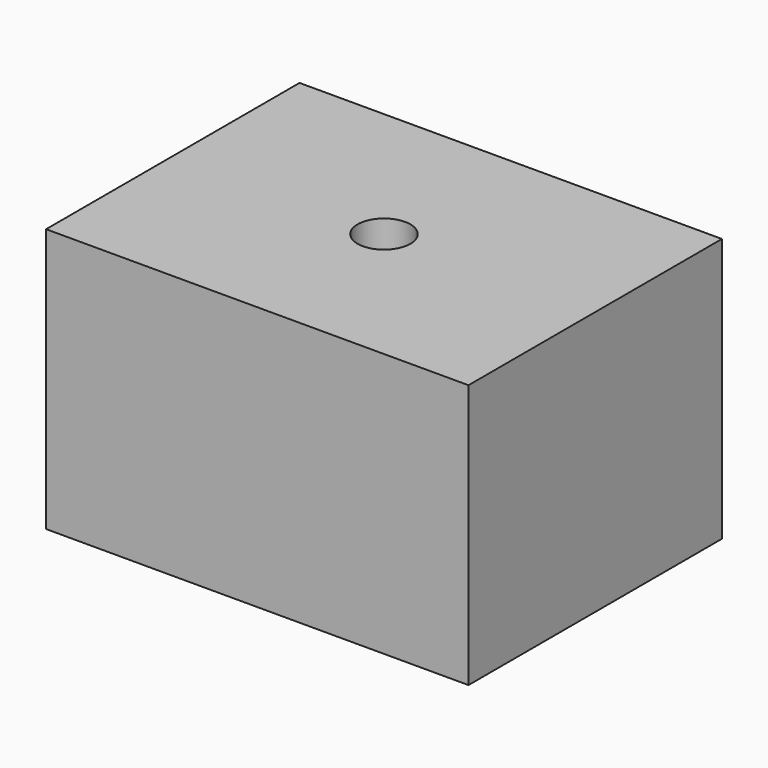
from build123d import *

# Parameters (mm, degrees)
F0_W     = 80
F0_H     = 60
F1_DEPTH = 50
F2_R     = 5
F3_DEPTH = 25


# Not quite as in the source:
# - a feature names something its author has since deleted; it is built from what else it names


with BuildPart() as f1:
    # F0 (on Top) → F1 (new body)
    with BuildSketch(Plane.XY):
        Rectangle(F0_W, F0_H)
    extrude(amount=F1_DEPTH)

    # F2 (on face) → F3 (cut)
    with BuildSketch(Plane.XY.offset(50)):
        Circle(F2_R)
    extrude(amount=-F3_DEPTH, mode=Mode.SUBTRACT)


solid = f1.part
